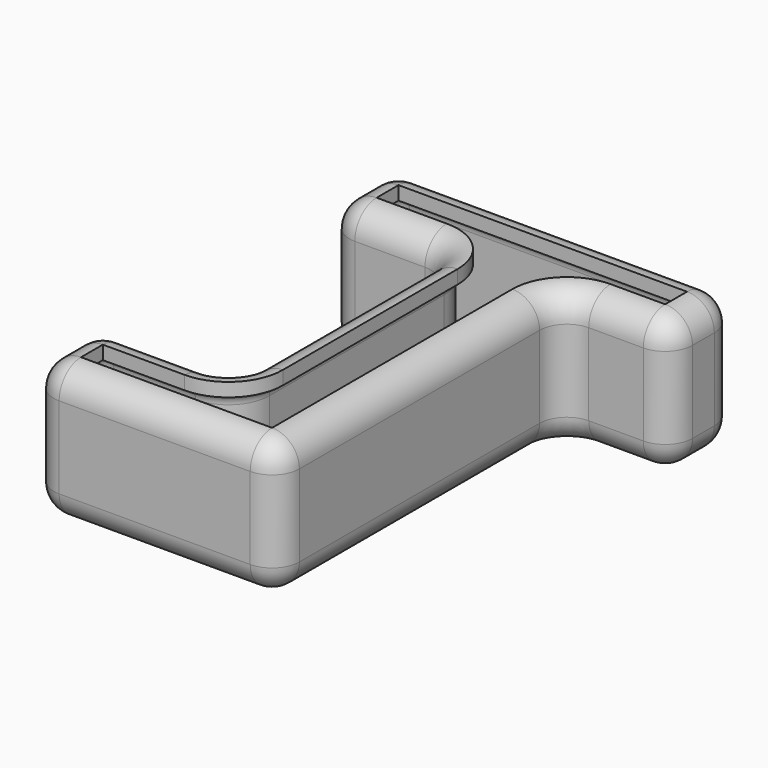
from build123d import *

# Parameters (mm, degrees)
F1_DEPTH = 25
F2_R     = 5
F3_T     = -2.5


# Not quite as in the source:
# - a shell that OpenCascade refuses in one call is made with other operations: the cavity is built on its own and cut out


with BuildPart() as f1:
    # F0 (on Top) → F1 (new body)
    with BuildSketch(Plane.XY):
        Polygon((-37.5918000937, -44.5486523956), (-12.5918000937, -44.5486523956), (7.4081999063, -44.5486523956), (7.4081999063, 20.4513476044), (27.4081999063, 20.4513476044), (27.4081999063, 35.4513476044), (-35.4375796765, 35.4513476044), (-35.4375796765, 20.4513476044), (-12.5918000937, 20.4513476044), (-12.5918000937, -29.5486523956), (-37.5918000937, -29.5486523956), align=None)
    extrude(amount=F1_DEPTH)

    # F2
    f2_edges = [f1.edges().sort_by_distance(p)[0] for p in [
        (-35.43758, 20.451348, 12.5),
        (-12.5918, 20.451348, 12.5),
        (-24.01469, 20.451348, 0),
        (-24.01469, 20.451348, 25),
        (7.4082, -44.548652, 12.5),
        (7.4082, 20.451348, 12.5),
        (7.4082, -12.048652, 0),
        (7.4082, -12.048652, 25),
        (-37.5918, -44.548652, 12.5),
        (-15.0918, -44.548652, 25),
        (-15.0918, -44.548652, 0),
        (-37.5918, -29.548652, 12.5),
        (-37.5918, -37.048652, 0),
        (-37.5918, -37.048652, 25),
        (-12.5918, -29.548652, 12.5),
        (-25.0918, -29.548652, 0),
        (-25.0918, -29.548652, 25),
        (-12.5918, -4.548652, 25),
        (17.4082, 20.451348, 25),
        (27.4082, 27.951348, 25),
        (-4.01469, 35.451348, 25),
        (-35.43758, 27.951348, 25),
        (27.4082, 35.451348, 12.5),
        (-35.43758, 35.451348, 12.5),
        (-4.01469, 35.451348, 0),
        (27.4082, 20.451348, 12.5),
        (27.4082, 27.951348, 0),
        (-12.5918, -4.548652, 0),
        (17.4082, 20.451348, 0),
        (-35.43758, 27.951348, 0),
    ]]
    fillet(f2_edges, radius=F2_R)

    # F3: a shell. OpenCascade refuses it in one call, so the cavity is built on its own and cut out:
    # the body offset inwards by the wall thickness, plus a prism from it out through each open face.
    f3_core = offset(f1.part, amount=F3_T, mode=Mode.PRIVATE)
    f3_exits = [f3_core.faces().sort_by_distance(p)[0] for p in [
        (-5.055266, -1.381038, 22.5),
    ]]
    add(f3_core, mode=Mode.SUBTRACT)
    extrude(f3_exits, amount=-F3_T, mode=Mode.SUBTRACT)


solid = f1.part
